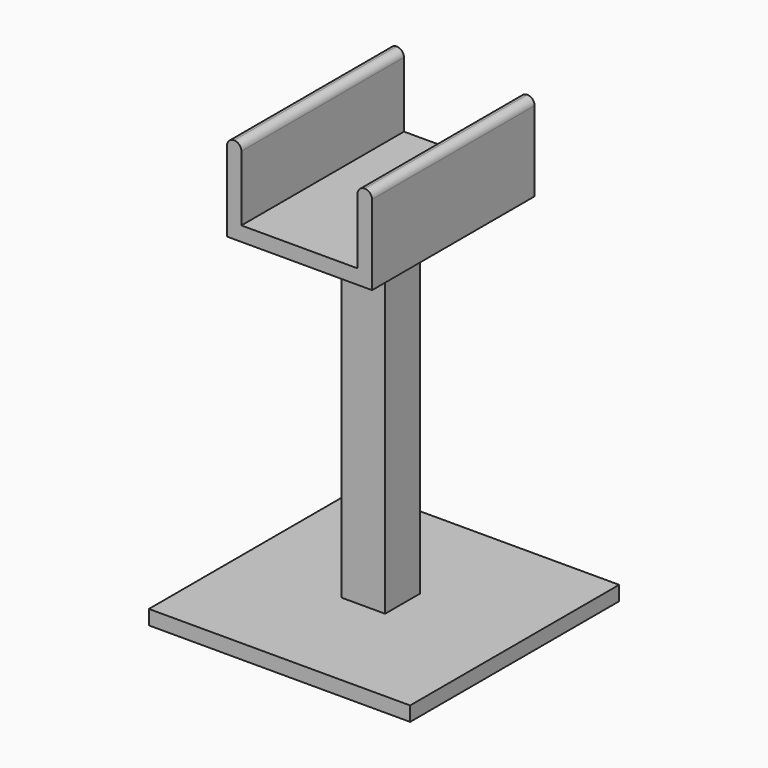
from build123d import *

# Parameters (mm, degrees)
F0_W     = 914.4
F0_H     = 914.4
F1_DEPTH = 50.8
F2_W     = 152.4
F2_H     = 152.4
F3_DEPTH = 1219.2
F4_W     = 508
F4_H     = 711.2
F5_DEPTH = 304.8
F6_W     = 406.4
F6_H     = 812.8
F7_DEPTH = 254
F8_R     = 25.39999


# Not quite as in the source:
# - a fillet or chamfer is up to 0.001 mm smaller than in the source, because OpenCascade refuses the exact size
# - a feature names something its author has since deleted; it is built from what else it names


with BuildPart() as f1:
    # F0 (on Top) → F1 (new body)
    with BuildSketch(Plane.XY):
        with Locations((11.3640455229, 0)):
            Rectangle(F0_W, F0_H)
    extrude(amount=F1_DEPTH)

    # F2 (on face) → F3 (join)
    with BuildSketch(Plane(origin=(0, 0, 0), x_dir=(1, 0, 0), z_dir=(0, 0, -1))):
        Rectangle(F2_W, F2_H)
    extrude(amount=-F3_DEPTH)

    # F4 (on face) → F5 (join)
    with BuildSketch(Plane.XY.offset(1219.2)):
        Rectangle(F4_W, F4_H)
    extrude(amount=F5_DEPTH)

    # F6 (on face) → F7 (cut)
    with BuildSketch(Plane.XY.offset(1524)):
        Rectangle(F6_W, F6_H)
    extrude(amount=-F7_DEPTH, mode=Mode.SUBTRACT)

    # F8 (radius 25.4 in the source; OpenCascade refuses exactly that, so slightly less here)
    f8_edges = [f1.edges().sort_by_distance(p)[0] for p in [
        (-254, 0, 1524),
        (-203.2, 0, 1524),
        (203.2, 0, 1524),
        (254, 0, 1524),
    ]]
    fillet(f8_edges, radius=F8_R)


solid = f1.part
